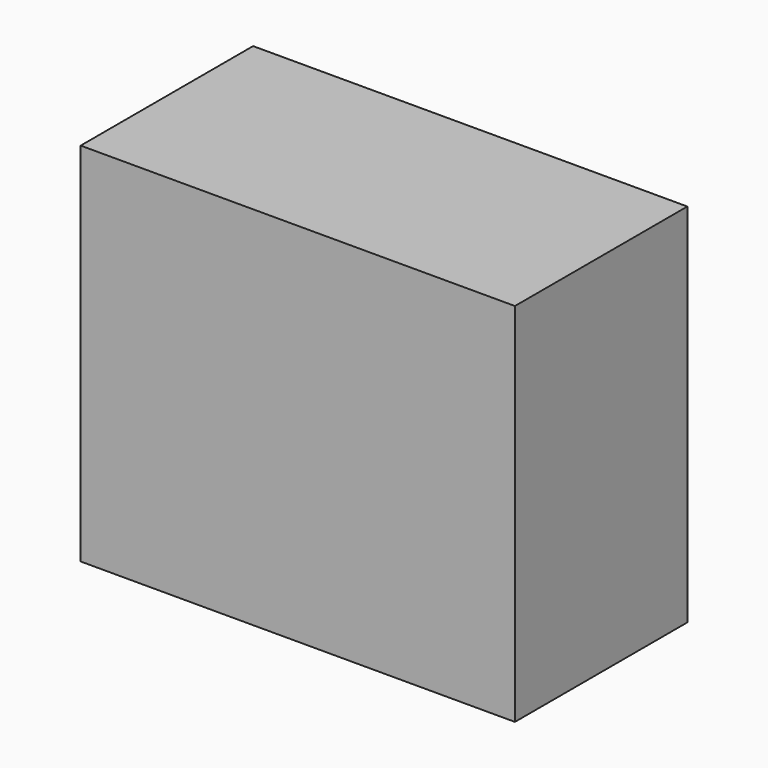
from build123d import *

# Parameters (mm, degrees)
F0_W     = 51.1811003089
F0_H     = 43.1526899338
F1_DEPTH = 25.4


# Not quite as in the source:
# - the program builds the solid bodies; features that only make, move or delete a surface that nothing else refers to are left out


with BuildPart() as f1:
    # F0 (on Front) → F1 (new body)
    with BuildSketch(Plane.XZ):
        with Locations((-85.3018276393, 30.1065295935)):
            Rectangle(F0_W, F0_H)
    extrude(amount=F1_DEPTH)


solid = f1.part
